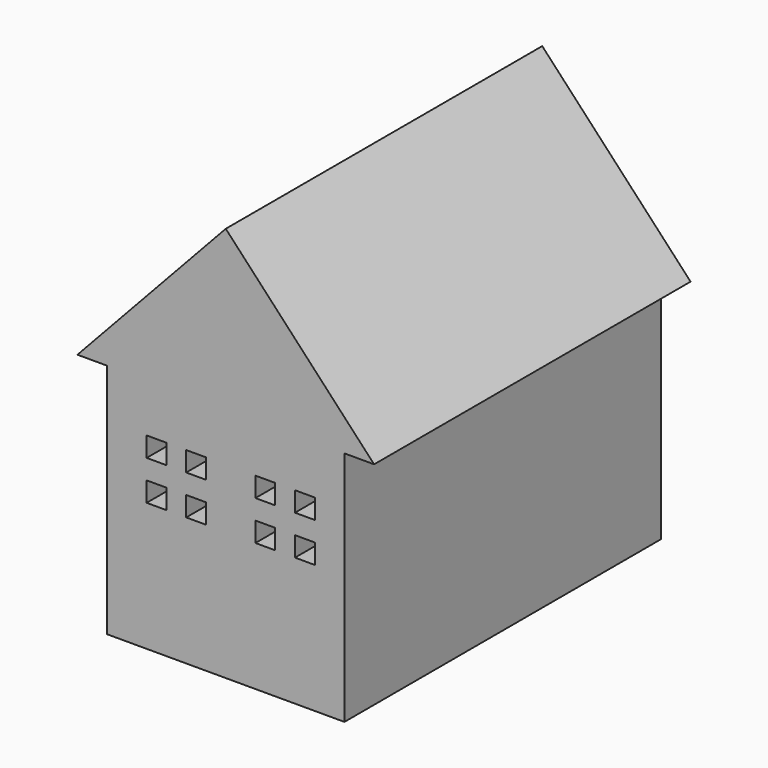
from build123d import *

# Parameters (mm, degrees)
F0_W     = 25.4
F0_H     = 25.4
F1_DEPTH = 25.4
F3_DEPTH = 25.4
F2_W     = 1.27
F2_H     = 1.27
F4_DEPTH = 25.4


# Not quite as in the source:
# - the program builds the solid bodies; features that only make, move or delete a surface that nothing else refers to are left out


with BuildPart() as f1:
    # F0 (on Front) → F1 (new body)
    with BuildSketch(Plane.XZ):
        with Locations((-12.7, 12.7)):
            Rectangle(F0_W, F0_H)
    extrude(amount=F1_DEPTH)

    # F2 (on face) → F3 (cut)
    with BuildSketch(Plane.XZ):
        Polygon((-3.9930980909, 15.1806421435), (-5.8980980909, 15.1806421435), (-5.8980980909, 0), (0, 0), (0, 25.4), (-13.5180980909, 25.4), align=None)
        Polygon((-25.4, 0), (-21.1380980909, 0), (-21.1380980909, 15.1806421435), (-23.0430980909, 15.1806421435), (-13.5180980909, 25.4), (-25.4, 25.4), align=None)
    extrude(amount=F3_DEPTH, mode=Mode.SUBTRACT)

    # F2 (on face) → F4 (cut)
    with BuildSketch(Plane.XZ):
        with Locations((-17.9630980909, 11.43)):
            Rectangle(F2_W, F2_H)
        with Locations((-17.9630980909, 8.89)):
            Rectangle(F2_W, F2_H)
        with Locations((-15.4230980909, 11.43)):
            Rectangle(F2_W, F2_H)
        with Locations((-15.4230980909, 8.89)):
            Rectangle(F2_W, F2_H)
        with Locations((-10.9780980909, 8.89)):
            Rectangle(F2_W, F2_H)
        with Locations((-8.4380980909, 8.89)):
            Rectangle(F2_W, F2_H)
        with Locations((-10.9780980909, 11.43)):
            Rectangle(F2_W, F2_H)
        with Locations((-8.4380980909, 11.43)):
            Rectangle(F2_W, F2_H)
    extrude(amount=F4_DEPTH, mode=Mode.SUBTRACT)


solid = f1.part
